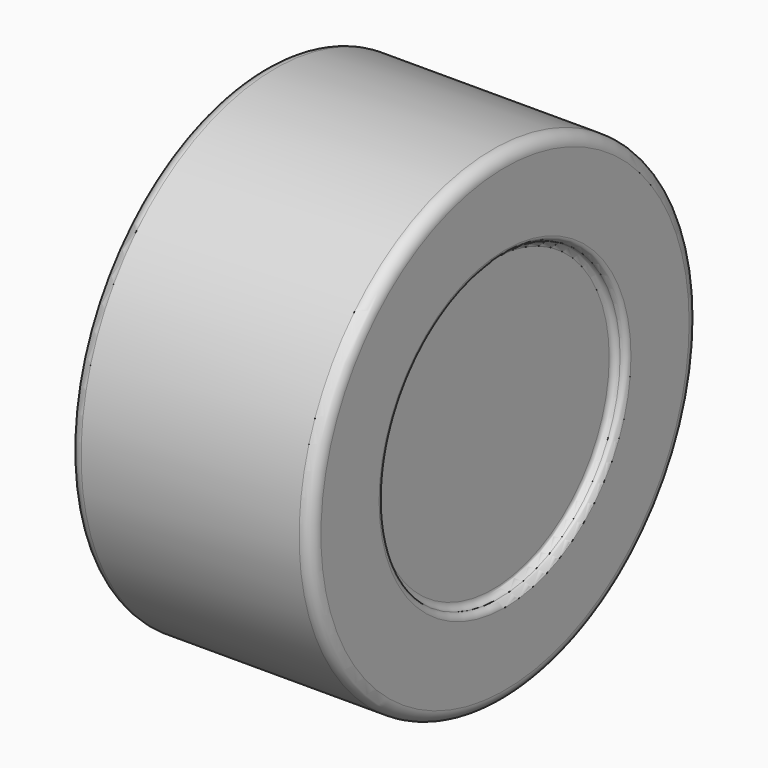
from build123d import *

# Parameters (mm, degrees)
F0_R      = 100
F1_DEPTH  = 100
F2_R      = 62.5
F3_DEPTH  = 50
F4_R      = 62.5
F5_DEPTH  = 5
F6_R      = 5
F7_R      = 37.5
F8_DEPTH  = 30
F9_R      = 10
F10_DEPTH = 25
F11_R     = 2.49999


# Not quite as in the source:
# - a fillet or chamfer is up to 0.001 mm smaller than in the source, because OpenCascade refuses the exact size


with BuildPart() as f1:
    # F0 (on Right) → F1 (new body)
    with BuildSketch(Plane.YZ):
        Circle(F0_R)
    extrude(amount=F1_DEPTH)

    # F2 (on face) → F3 (cut)
    with BuildSketch(Plane(origin=(0, 0, 0), x_dir=(0, -1, 0), z_dir=(-1, 0, 0))):
        Circle(F2_R)
    extrude(amount=-F3_DEPTH, mode=Mode.SUBTRACT)

    # F4 (on face) → F5 (cut)
    with BuildSketch(Plane.YZ.offset(100)):
        Circle(F4_R)
    extrude(amount=-F5_DEPTH, mode=Mode.SUBTRACT)

    # F6
    f6_edges = [f1.edges().sort_by_distance(p)[0] for p in [
        (0, -100, 0),
        (100, -100, 0),
    ]]
    fillet(f6_edges, radius=F6_R)

    # F7 (on face) → F8 (join)
    with BuildSketch(Plane(origin=(50, 0, 0), x_dir=(0, -1, 0), z_dir=(-1, 0, 0))):
        Circle(F7_R)
    extrude(amount=F8_DEPTH)

    # F9 (on face) → F10 (cut)
    with BuildSketch(Plane(origin=(20, 0, 0), x_dir=(0, -1, 0), z_dir=(-1, 0, 0))):
        Circle(F9_R)
    extrude(amount=-F10_DEPTH, mode=Mode.SUBTRACT)

    # F11 (radius 2.5 in the source; OpenCascade refuses exactly that, so slightly less here)
    f11_edges = [f1.edges().sort_by_distance(p)[0] for p in [
        (0, 62.5, 0),
        (50, 62.5, 0),
        (50, 37.5, 0),
        (20, 37.5, 0),
        (100, -62.5, 0),
        (95, -62.5, 0),
    ]]
    fillet(f11_edges, radius=F11_R)


solid = f1.part
